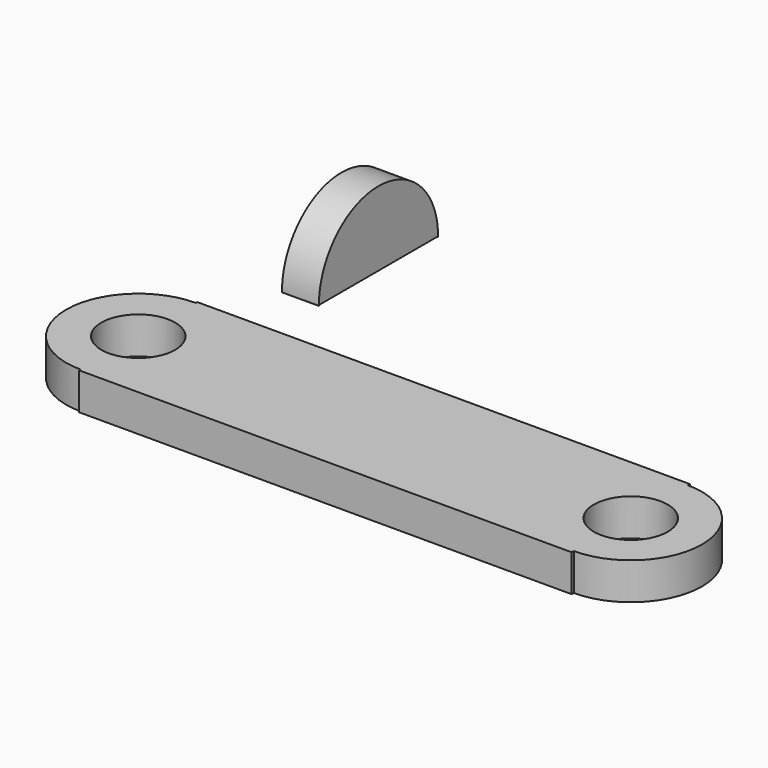
from build123d import *

# Parameters (mm, degrees)
F0_R     = 9.525
F1_DEPTH = 9.525
F3_DEPTH = 9.525


with BuildPart() as f1:
    # F0 (on Top) → F1 (new body)
    with BuildSketch(Plane.XY):
        with BuildLine():
            Line((-52.308280021, 0.4681994029), (-52.308280021, 0))
            Line((-52.308280021, 0), (74.691719979, 0))
            Line((74.691719979, 0), (74.691719979, 0.6744954629))
            ThreePointArc((74.691719979, 0.6744954629), (93.0672245161, 19.05), (74.691719979, 37.4255045371))
            Line((74.691719979, 37.4255045371), (74.691719979, 38.1))
            Line((74.691719979, 38.1), (-52.308280021, 38.1))
            Line((-52.308280021, 38.1), (-52.308280021, 37.6318005971))
            ThreePointArc((-52.308280021, 37.6318005971), (-70.890080618, 19.05), (-52.308280021, 0.4681994029))
        make_face()
        with Locations((-52.308280021, 19.05)):
            Circle(F0_R, mode=Mode.SUBTRACT)
        with Locations((74.691719979, 19.05)):
            Circle(F0_R, mode=Mode.SUBTRACT)
    extrude(amount=F1_DEPTH)


with BuildPart() as f3:
    # F2 (on Right) → F3 (new body)
    with BuildSketch(Plane.YZ):
        with BuildLine():
            ThreePointArc((38.3800417185, 44.2407319942), (19.1900208592, 63.6411618636), (0, 44.2407319942))
            Line((0, 44.2407319942), (0, 44.45))
            Line((0, 44.45), (38.3800417185, 44.45))
            Line((38.3800417185, 44.45), (38.3800417185, 44.2407319942))
        make_face()
    extrude(amount=F3_DEPTH)


solid = Compound([f1.part, f3.part])
